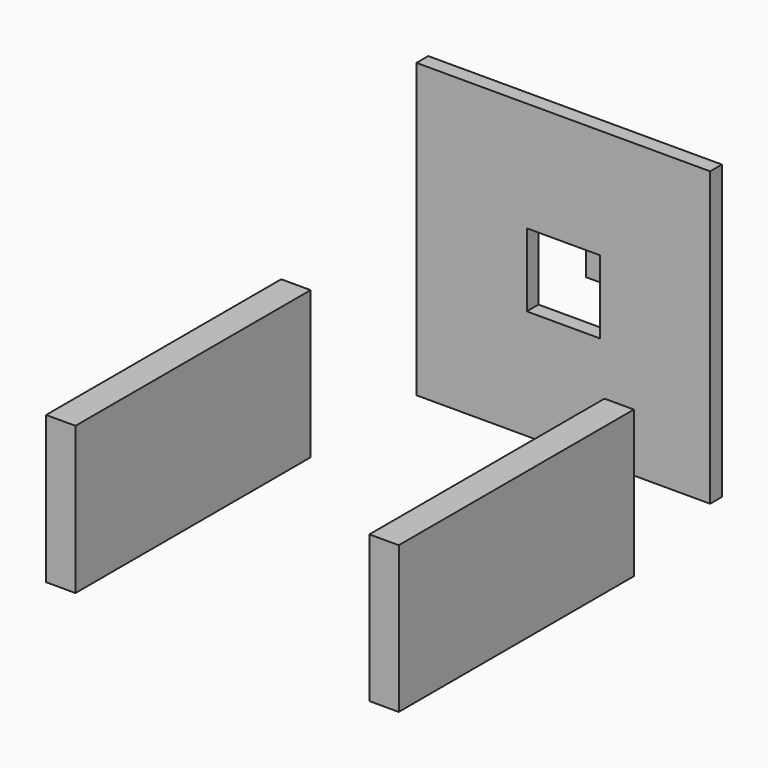
from build123d import *

# Parameters (mm, degrees)
F1_W      = 609.1041564941
F1_H      = 607.0808172226
F1_W_2    = 151.7698764801
F1_H_2    = 151.7701148987
F2_DEPTH  = 30.48
F7_E6_W   = 305.4414391518
F7_E6_H   = 609.6
F8_DEPTH  = 30.48
F7_E7_W   = 304.4300079346
F7_E7_H   = 609.6
F9_DEPTH  = 30.48
F12_W     = 150.6595611572
F12_H     = 150.3119468689
F13_DEPTH = 30.48


# Not quite as in the source:
# - a feature of the source that left no trace in its solid (it failed there, or was rolled back) is left out
# - a pattern or mirror of a feature is missing from the dataset's text; its kind, count and spacing are read off the source's solid
# - the program builds the solid bodies; features that only make, move or delete a surface that nothing else refers to are left out


with BuildPart() as f2:
    # F1 (on offset) → F2 (new body)
    with BuildSketch(Plane.XZ.offset(-914.4)):
        Rectangle(F1_W, F1_H)
        Rectangle(F1_W_2, F1_H_2, mode=Mode.SUBTRACT)
    extrude(amount=F2_DEPTH)


with BuildPart() as f8:
    # F7_E6 (on explicit) → F8 (new body)
    with BuildSketch(Plane(origin=(-304.8, 0, -305.4414391518), x_dir=(0, 0, 1), z_dir=(-1, 0, 0))):
        with Locations((152.7207195759, 304.8)):
            Rectangle(F7_E6_W, F7_E6_H)
    extrude(amount=F8_DEPTH)

    # F8_copies: F8 across plane


with BuildPart() as f8_1:
    add(f8.part)
    add(f8.part.mirror(Plane(origin=(-335.28, 0, 0), x_dir=(0, 0, -1), z_dir=(-1, 0, 0))))


with BuildPart() as f9:
    # F7_E7 (on explicit) → F9 (new body)
    with BuildSketch(Plane(origin=(304.8, 0, 0), x_dir=(0, 0, -1), z_dir=(1, 0, 0))):
        with Locations((152.2150039673, 304.8)):
            Rectangle(F7_E7_W, F7_E7_H)
    extrude(amount=F9_DEPTH)

    # F9_copies: F9 across plane


with BuildPart() as f9_1:
    add(f9.part)
    add(f9.part.mirror(Plane(origin=(335.28, 0, 0), x_dir=(0, 0, 1), z_dir=(1, 0, 0))))


with BuildPart() as f13:
    # F12 (on offset) → F13 (new body)
    with BuildSketch(Plane.XZ.offset(-1066.8)):
        Rectangle(F12_W, F12_H)
    extrude(amount=F13_DEPTH)


solid = Compound([f2.part, f8_1.part, f9_1.part, f13.part])
